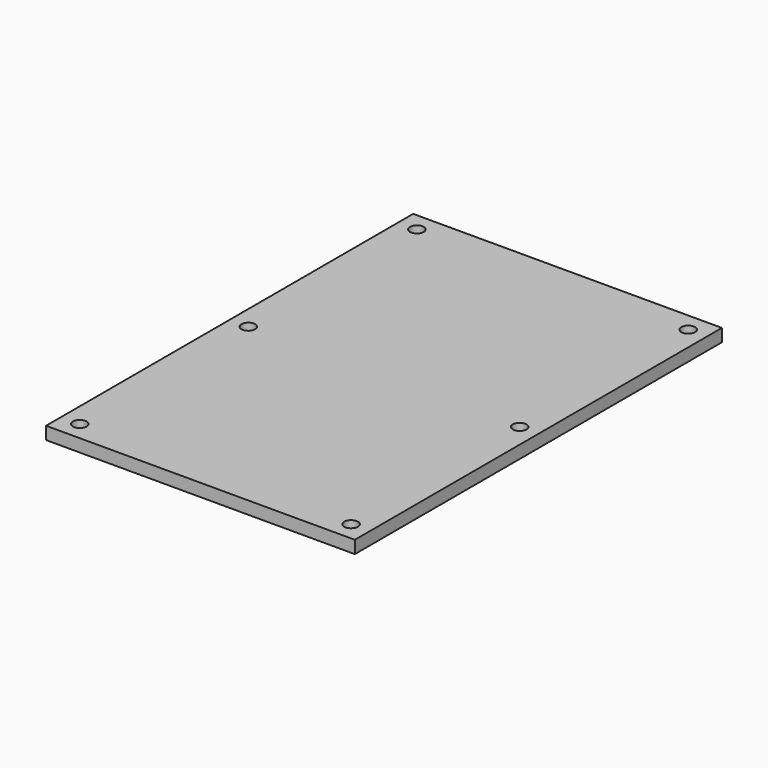
from build123d import *

# Parameters (mm, degrees)
F0_W     = 77.47
F0_H     = 115.1382
F1_DEPTH = 3.175
F3_D     = 3.4544


# Not quite as in the source:
# - a length typed as a fraction of an inch, garbled in the dataset ("3 / 203.2 mm" for 3/8 in), is restored


with BuildPart() as f1:
    # F0 (on Top) → F1 (new body)
    with BuildSketch(Plane.XY):
        Rectangle(F0_W, F0_H)
    extrude(amount=F1_DEPTH)

    # F3 (through all)
    with Locations(Plane.XY.offset(3.175)):
        with Locations((-34.036, 52.8701), (34.036, 52.8701), (34.036, -52.8701), (-34.036, -52.8701), (-34.036, 0), (34.036, 0)):
            Hole(F3_D / 2)


solid = f1.part
